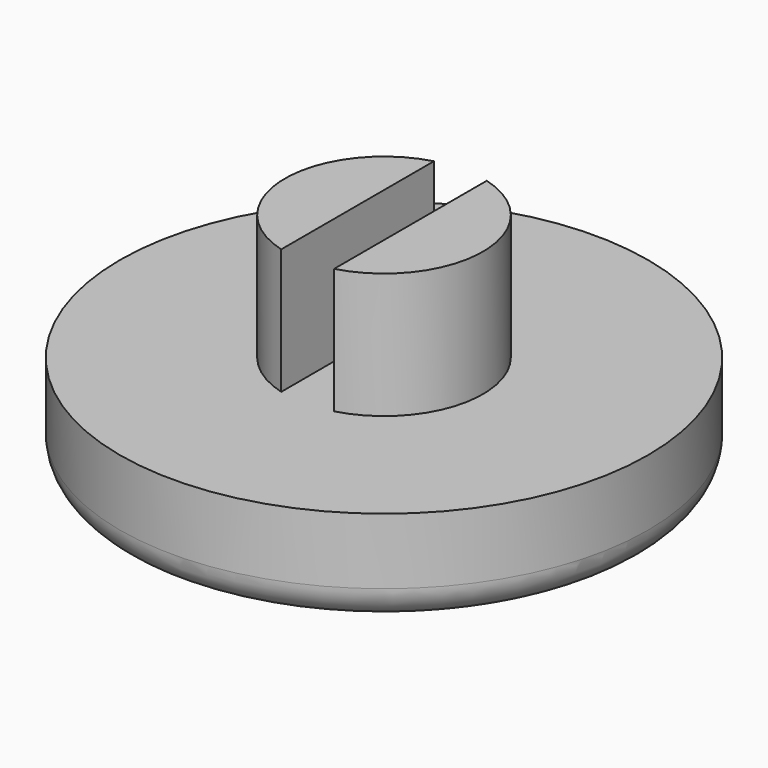
from build123d import *

# Parameters (mm, degrees)
F0_R     = 4
F1_DEPTH = 1.5
F2_R     = 1.5
F3_DEPTH = 1.9
F5_DEPTH = 1.9
F7_DEPTH = 0.3
F8_R     = 0.5


# Not quite as in the source:
# - a feature names something its author has since deleted; it is built from what else it names


with BuildPart() as f1:
    # F0 (on Top) → F1 (new body)
    with BuildSketch(Plane.XY):
        Circle(F0_R)
    extrude(amount=F1_DEPTH)

    # F2 (on face) → F3 (join)
    with BuildSketch(Plane.XY.offset(1.5)):
        Circle(F2_R)
    extrude(amount=F3_DEPTH)

    # F4 (on face) → F5 (cut)
    with BuildSketch(Plane.XY.offset(3.4)):
        with BuildLine():
            ThreePointArc((-0.4, -1.4456832295), (0, -1.5), (0.4, -1.4456832295))
            Line((0.4, -1.4456832295), (0.4, 1.4456832295))
            ThreePointArc((0.4, 1.4456832295), (0, 1.5), (-0.4, 1.4456832295))
            Line((-0.4, 1.4456832295), (-0.4, -1.4456832295))
        make_face()
        with BuildLine():
            ThreePointArc((-0.4, 1.4456832295), (0, 1.5), (0.4, 1.4456832295))
            Line((0.4, 1.4456832295), (0.4, 2.5026321411))
            Line((0.4, 2.5026321411), (-0.4, 2.5026321411))
            Line((-0.4, 2.5026321411), (-0.4, 1.4456832295))
        make_face()
    extrude(amount=-F5_DEPTH, mode=Mode.SUBTRACT)

    # F6 (on face) → F7 (join)
    with BuildSketch(Plane.XY.offset(1.5)):
        with BuildLine():
            ThreePointArc((0.4, 1.3937359865), (1.1581234822, 0.8724964183), (1.45, 0))
            ThreePointArc((1.45, 0), (1.1581234822, -0.8724964183), (0.4, -1.3937359865))
            Line((0.4, -1.3937359865), (0.4, -1.4456832295))
            ThreePointArc((0.4, -1.4456832295), (1.5, 0), (0.4, 1.4456832295))
            Line((0.4, 1.4456832295), (0.4, 1.3937359865))
        make_face()
        with BuildLine():
            ThreePointArc((-0.4, -1.3937359865), (-1.45, 0), (-0.4, 1.3937359865))
            Line((-0.4, 1.3937359865), (-0.4, 1.4456832295))
            ThreePointArc((-0.4, 1.4456832295), (-1.5, 0), (-0.4, -1.4456832295))
            Line((-0.4, -1.4456832295), (-0.4, -1.3937359865))
        make_face()
    extrude(amount=F7_DEPTH)

    # F8
    f8_edges = [f1.edges().sort_by_distance(p)[0] for p in [
        (-4, 0, 0),
    ]]
    fillet(f8_edges, radius=F8_R)


solid = f1.part
